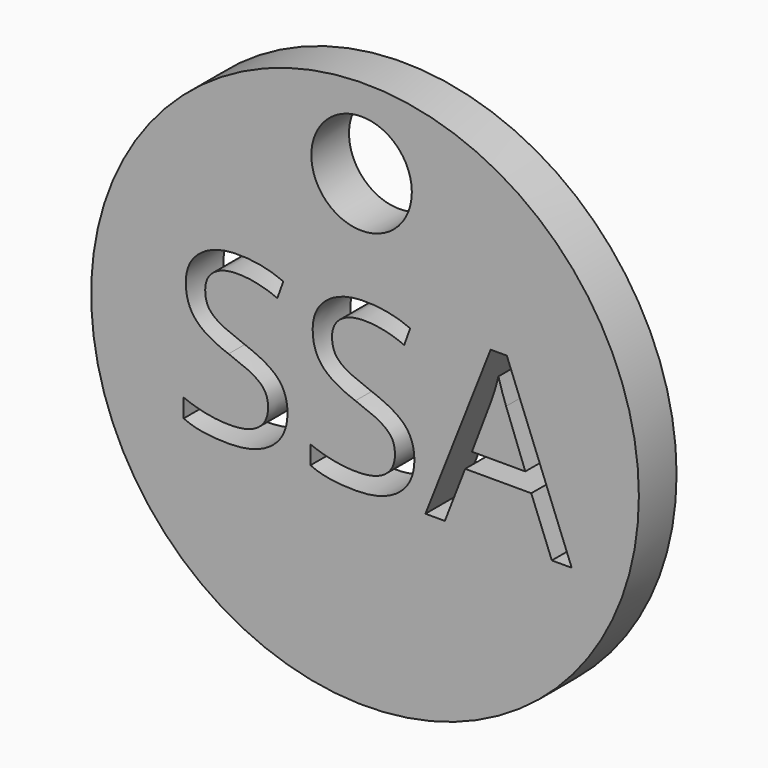
from build123d import *

# Parameters (mm, degrees)
F0_R         = 17.715109064
F1_DEPTH     = 3.048
F2_TEXT_SIZE = 14.9503389063
F3_DEPTH     = 25.4
F4_DEPTH     = 1.016
F5_R         = 3.2509958561
F6_DEPTH     = 3.81


# Not quite as in the source:
# - Text() gives the source's letters only with a copy of the font that has no kerning and outlines rounded to 1/6400 em; it was checked with that copy


with BuildPart() as f1:
    # F0 (on Front) → F1 (new body)
    with BuildSketch(Plane.XZ):
        with Locations((-12.2650060803, -15.1396170259)):
            Circle(F0_R)
    extrude(amount=F1_DEPTH)

    # F2 (on face) → F3 (cut)
    with BuildSketch(Plane.XZ.offset(3.048)):
        with Locations((-24.770242162, -20.640000701)):
            Text('SSA', F2_TEXT_SIZE, font='Open Sans', text_align=(TextAlign.LEFT, TextAlign.BOTTOM))
    extrude(amount=-F3_DEPTH, mode=Mode.SUBTRACT)

    # F2 (on face) → F4 (cut)
    with BuildSketch(Plane.XZ.offset(3.048)):
        with Locations((-24.770242162, -20.640000701)):
            Text('SSA', F2_TEXT_SIZE, font='Open Sans', text_align=(TextAlign.LEFT, TextAlign.BOTTOM))
    extrude(amount=-F4_DEPTH, mode=Mode.SUBTRACT)

    # F5 (on Front) → F6 (cut)
    with BuildSketch(Plane.XZ):
        with Locations((-12.4879488721, -2.6137568057)):
            Circle(F5_R)
    extrude(amount=F6_DEPTH, mode=Mode.SUBTRACT)


solid = f1.part
